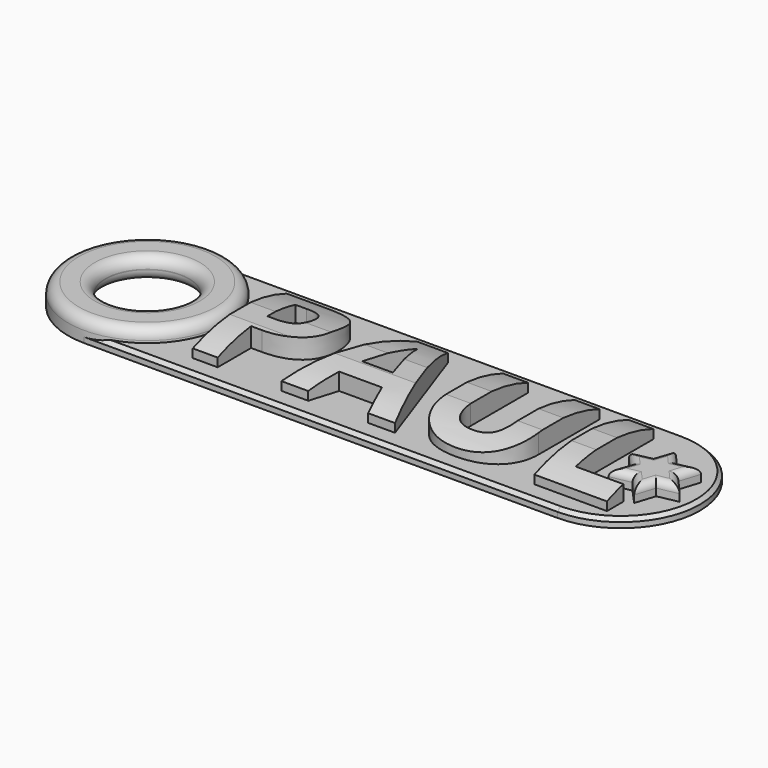
from build123d import *

# Parameters (mm, degrees)
F0_R          = 5.8386807056
F1_DEPTH      = 1.25
F2_TEXT_SIZE  = 23.0094133359
F3_DEPTH      = 4
F5_DEPTH      = 50
F6_R          = 11.0439514966
F6_R_2        = 5.8386807056
F7_DEPTH      = 1.8
F8_R          = 1.49
F10_DEPTH     = 2
F11_R         = 1
F12_T4_DEPTH  = 70.0027790623
F12_S5_R      = 11.0439514966
F12_T6_DEPTH  = 37
F12_T8_ANGLE  = 180
F12_T12_DEPTH = 70.0027790623
F12_S13_R     = 11.0439514966
F12_T14_DEPTH = 37


# Not quite as in the source:
# - a fillet or chamfer that OpenCascade refuses, or shapes differently, is made with other operations: its cross-section is extruded or revolved along the edge and cut away or added
# - Text() gives the source's letters only with a copy of the font that has no kerning and outlines rounded to 1/6400 em; it was checked with that copy


with BuildPart() as f1:
    # F0 (on Top) → F1 (new body)
    with BuildSketch(Plane.XY):
        with BuildLine():
            Line((29.4512491673, 11.0439514966), (-36.694005413, 11.0439514966))
            ThreePointArc((-36.694005413, 11.0439514966), (-47.7379569096, 0), (-36.694005413, -11.0439514966))
            Line((-36.694005413, -11.0439514966), (29.4512491673, -11.0439514966))
            ThreePointArc((29.4512491673, -11.0439514966), (40.4952006639, 0), (29.4512491673, 11.0439514966))
        make_face()
        with Locations((-36.694005413, 0)):
            Circle(F0_R, mode=Mode.SUBTRACT)
    extrude(amount=F1_DEPTH)

    # F2 (on Top) → F3 (join)
    with BuildSketch(Plane.XY):
        with Locations((-25.7921982557, -8.2833888009)):
            Text('PAUL', F2_TEXT_SIZE, font='Open Sans', font_style=FontStyle.BOLD, text_align=(TextAlign.LEFT, TextAlign.BOTTOM))
    extrude(amount=F3_DEPTH)

    # F4 (on Right) → F5 (cut, symmetric)
    with BuildSketch(Plane.YZ):
        with BuildLine():
            ThreePointArc((-9.021110195, 2.1300164517), (0, 4.0756319036), (9.021110195, 2.1300164517))
            Line((9.021110195, 2.1300164517), (9.021110195, 6.5328008495))
            Line((9.021110195, 6.5328008495), (-9.4408150762, 6.5328008495))
            Line((-9.4408150762, 6.5328008495), (-9.021110195, 2.1300164517))
        make_face()
    extrude(amount=F5_DEPTH, both=True, mode=Mode.SUBTRACT)

    # F6 (on face) → F7 (join)
    with BuildSketch(Plane.XY.offset(1.25)):
        with Locations((-36.694005413, 0)):
            Circle(F6_R)
        with Locations((-36.694005413, 0)):
            Circle(F6_R_2, mode=Mode.SUBTRACT)
    extrude(amount=F7_DEPTH)

    # F8
    f8_edges = [f1.edges().sort_by_distance(p)[0] for p in [
        (-47.737957, 0, 3.05),
        (-42.532686, 0, 3.05),
        (-42.532686, 0, 0),
    ]]
    fillet(f8_edges, radius=F8_R)

    # F9 (on face) → F10 (join)
    with BuildSketch(Plane.XY.offset(1.25)):
        Polygon((35.1081187965, 2.7863767464), (33.2060886957, 4.9560660867), (32.2576394376, 2.1637850245), align=None)
        Polygon((37.927017729, 3.4020707822), (35.1081187965, 2.7863767464), (37.031457544, 0.5923801443), align=None)
        Polygon((37.031457544, 0.5923801443), (35.1081187965, 2.7863767464), (32.2576394376, 2.1637850245), (31.3192520181, -0.598873492), (33.283671945, -2.7561651688), (36.145398112, -2.1875032544), align=None)
        Polygon((31.3192520181, -0.598873492), (32.2576394376, 2.1637850245), (29.3765958759, 1.5345175763), align=None)
        Polygon((38.9754192494, -1.6251415385), (37.031457544, 0.5923801443), (36.145398112, -2.1875032544), align=None)
        Polygon((33.283671945, -2.7561651688), (31.3192520181, -0.598873492), (30.3912609816, -3.3309245482), align=None)
        Polygon((35.2691553217, -4.9365883586), (36.145398112, -2.1875032544), (33.283671945, -2.7561651688), align=None)
    extrude(amount=F10_DEPTH)

    # F11
    f11_edges = [f1.edges().sort_by_distance(p)[0] for p in [
        (34.157104, 3.871221, 3.25),
        (32.731864, 3.559926, 3.25),
        (30.817118, 1.849151, 3.25),
        (30.347924, 0.467822, 3.25),
        (30.855256, -1.964899, 3.25),
        (31.837466, -3.043545, 3.25),
        (34.276414, -3.846377, 3.25),
        (35.707277, -3.562046, 3.25),
        (37.560409, -1.906322, 3.25),
        (38.003438, -0.516381, 3.25),
        (37.479238, 1.997225, 3.25),
        (36.517568, 3.094224, 3.25),
    ]]
    fillet(f11_edges, radius=F11_R)

    # F12: chamfer of 0.5 on 1 edges, made by hand


with BuildPart() as f12_tool2:
    # F12_s3 → F12_t4 (new body)
    with BuildSketch(Plane.YZ.offset(-40.551529895)):
        Polygon((-10.5439514966, 1.25), (-11.0439514966, 0.75), (-11.0439514966, 1.25), align=None)
    extrude(amount=F12_T4_DEPTH)

    # F12_s5 → F12_t6 (cut, symmetric)
    with BuildSketch(Plane.XY.offset(1)):
        with Locations((-36.694005413, 0)):
            Circle(F12_S5_R)
    extrude(amount=F12_T6_DEPTH, both=True, mode=Mode.SUBTRACT)


with BuildPart() as f1_1:
    add(f1.part)

    # F12_t1: cut F12_tool2
    add(f12_tool2.part, mode=Mode.SUBTRACT)

    # F12_s7 → F12_t8 (revolve, cut)
    with BuildSketch(Plane.YZ.offset(29.4512491673)):
        Polygon((-10.5439514966, 1.25), (-11.0439514966, 0.75), (-11.0439514966, 1.25), align=None)
    revolve(axis=Axis((29.4512491673, 0, 1.25), (0, 0, 1)), revolution_arc=F12_T8_ANGLE, mode=Mode.SUBTRACT)


with BuildPart() as f12_tool10:
    # F12_s11 → F12_t12 (new body)
    with BuildSketch(Plane.YZ.offset(29.4512491673)):
        Polygon((10.5439514966, 1.25), (11.0439514966, 0.75), (11.0439514966, 1.25), align=None)
    extrude(amount=-F12_T12_DEPTH)

    # F12_s13 → F12_t14 (cut, symmetric)
    with BuildSketch(Plane.XY.offset(1)):
        with Locations((-36.694005413, 0)):
            Circle(F12_S13_R)
    extrude(amount=F12_T14_DEPTH, both=True, mode=Mode.SUBTRACT)


with BuildPart() as f1_2:
    add(f1_1.part)

    # F12_t9: cut F12_tool10
    add(f12_tool10.part, mode=Mode.SUBTRACT)


solid = f1_2.part
